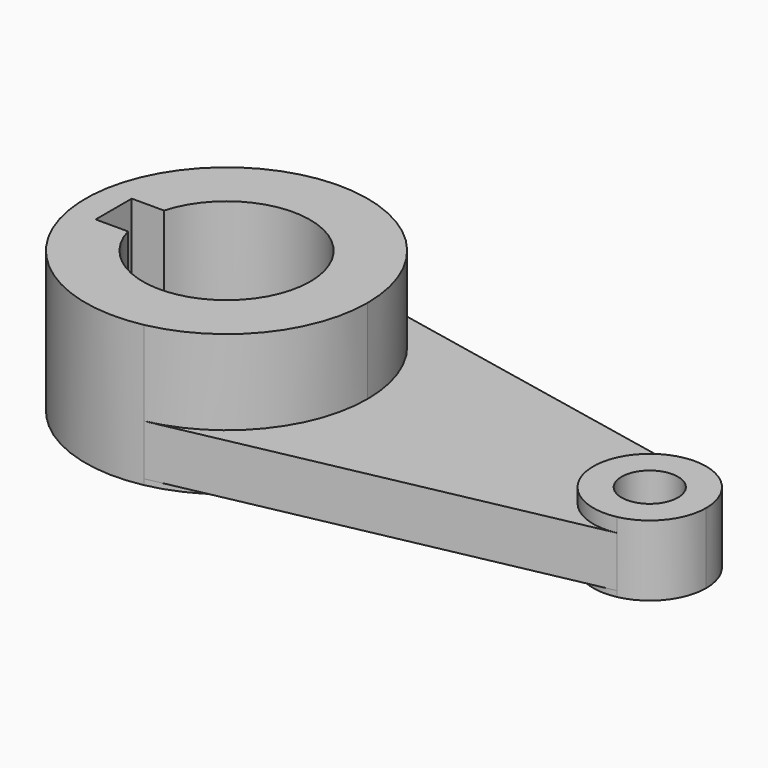
from build123d import *

# Parameters (mm, degrees)
F1_DEPTH  = 50
F2_DEPTH  = 25
F3_DEPTH  = 20
F4_DEPTH  = 2
F5_R      = 29.64758
F6_DEPTH  = 130
F7_W      = 22.106876
F7_H      = 16
F8_DEPTH  = 118
F9_R      = 10
F10_DEPTH = 52


with BuildPart() as f1:
    # F0 (on Top) → F1 (new body)
    with BuildSketch(Plane.XY):
        with BuildLine():
            ThreePointArc((10, -48.989795), (38.729833, -31.622777), (50, 0))
            ThreePointArc((50, 0), (38.729833, 31.622777), (10, 48.989795))
            ThreePointArc((10, 48.989795), (-50, 0), (10, -48.989795))
        make_face()
    extrude(amount=F1_DEPTH)



with BuildPart() as f2:
    # F0 (on Top) → F2 (new body)
    with BuildSketch(Plane.XY):
        with BuildLine():
            ThreePointArc((170, 0), (165.491933, 12.649111), (154, 19.595918))
            ThreePointArc((154, 19.595918), (130, 0), (154, -19.595918))
            ThreePointArc((154, -19.595918), (165.491933, -12.649111), (170, 0))
        make_face()
    extrude(amount=F2_DEPTH)


with BuildPart() as f1_1:
    add(f1.part)

    add(f2.part)  # F3 merges F2
    # F0 (on Top) → F3 (join)
    with BuildSketch(Plane.XY):
        with BuildLine():
            ThreePointArc((10, 48.989795), (38.729833, 31.622777), (50, 0))
            ThreePointArc((50, 0), (38.729833, -31.622777), (10, -48.989795))
            Line((10, -48.989795), (154, -19.595918))
            ThreePointArc((154, -19.595918), (130, 0), (154, 19.595918))
            Line((154, 19.595918), (10, 48.989795))
        make_face()
    extrude(amount=F3_DEPTH)

    # F0 (on Top) → F4 (cut)
    with BuildSketch(Plane.XY):
        with BuildLine():
            ThreePointArc((10, 48.989795), (38.729833, 31.622777), (50, 0))
            ThreePointArc((50, 0), (38.729833, -31.622777), (10, -48.989795))
            Line((10, -48.989795), (154, -19.595918))
            ThreePointArc((154, -19.595918), (130, 0), (154, 19.595918))
            Line((154, 19.595918), (10, 48.989795))
        make_face()
    extrude(amount=F4_DEPTH, mode=Mode.SUBTRACT)

    # F5 (on face) → F6 (cut)
    with BuildSketch(Plane.XY.offset(50)):
        Circle(F5_R)
    extrude(amount=-F6_DEPTH, mode=Mode.SUBTRACT)

    # F7 (on face) → F8 (cut)
    with BuildSketch(Plane.XY.offset(50)):
        with Locations((-28.946562, 0)):
            Rectangle(F7_W, F7_H)
    extrude(amount=-F8_DEPTH, mode=Mode.SUBTRACT)

    # F9 (on face) → F10 (cut)
    with BuildSketch(Plane.XY.offset(25)):
        with Locations((150, 0)):
            Circle(F9_R)
    extrude(amount=-F10_DEPTH, mode=Mode.SUBTRACT)


solid = f1_1.part
